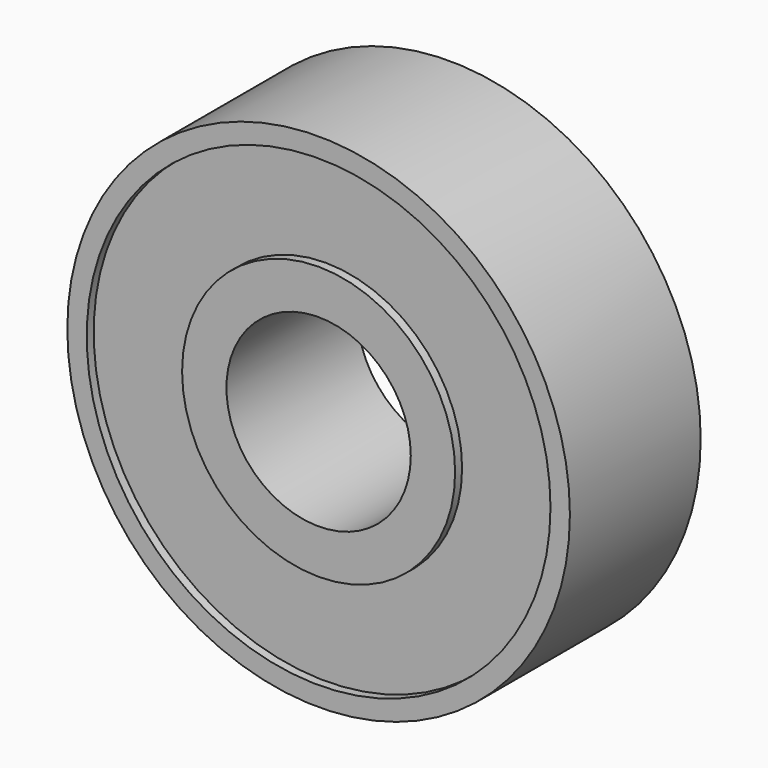
from build123d import *

# Parameters (mm, degrees)
F0_R     = 11.0109
F0_R_2   = 5.969
F1_DEPTH = 3.5814
F2_R     = 10.16
F2_R_2   = 5.9817
F3_DEPTH = 0.381
F4_R     = 5.969
F4_R_2   = 4.0386
F5_DEPTH = 3.5814


# Not quite as in the source:
# - a pattern or mirror of a feature is missing from the dataset's text; its kind, count and spacing are read off the source's solid


with BuildPart() as f1:
    # F0 (on Front) → F1 (new body, symmetric)
    with BuildSketch(Plane.XZ):
        Circle(F0_R)
        Circle(F0_R_2, mode=Mode.SUBTRACT)
    extrude(amount=F1_DEPTH, both=True)

    # F2 (on face) → F3 (cut)
    with BuildSketch(Plane.XZ.offset(3.5814)):
        Circle(F2_R)
        Circle(F2_R_2, mode=Mode.SUBTRACT)
    f3 = extrude(amount=-F3_DEPTH, mode=Mode.SUBTRACT)

    # F3_copies: F3 across plane
    add(f3.mirror(Plane.ZX), mode=Mode.SUBTRACT)

    # F4 (on Front) → F5 (join, symmetric)
    with BuildSketch(Plane.XZ):
        Circle(F4_R)
        Circle(F4_R_2, mode=Mode.SUBTRACT)
    extrude(amount=F5_DEPTH, both=True)


solid = f1.part
